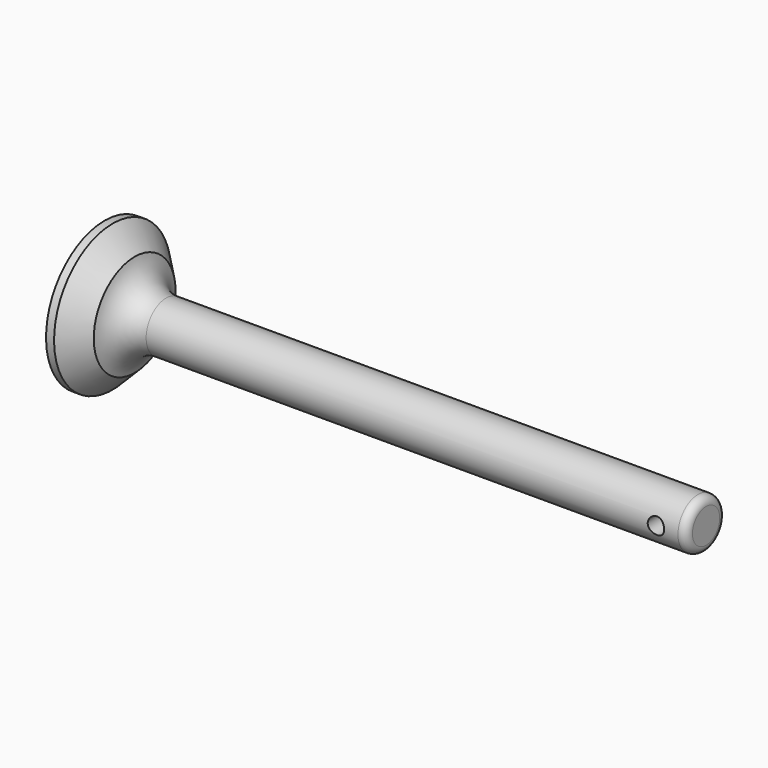
from build123d import *

# Parameters (mm, degrees)
F3_R     = 0.508
F6_R     = 0.5207
F7_DEPTH = 9.7165


# Not quite as in the source:
# - a fillet or chamfer that OpenCascade refuses, or shapes differently, is made with other operations: its cross-section is extruded or revolved along the edge and cut away or added


with BuildPart() as f1:
    # F0 (on Front) → F1 (revolve)
    with BuildSketch(Plane.XZ):
        Polygon((0, 4.6355), (0, 0), (38.1, 0), (38.1, 1.5875), (1.905, 1.5875), (1.905, 3.2385), (0.508, 4.6355), align=None)
    revolve(axis=Axis((19.05, 0, 0), (1, 0, 0)))

    # F2: fillet of radius 2.032 on 1 edges, made by hand

    # F2_s1 → F2_t2 (revolve)
    with BuildSketch(Plane.XZ):
        with BuildLine():
            ThreePointArc((1.905, 3.2385), (2.6058107165, 2.0537388432), (3.900961673, 1.5875))
            Line((3.900961673, 1.5875), (3.900961673, 1.54686))
            Line((3.900961673, 1.54686), (1.905, 1.54686))
            Line((1.905, 1.54686), (1.86436, 1.5875))
            ThreePointArc((1.86436, 1.5875), (1.86436, 2.413), (1.8650807665, 3.23088))
            Line((1.8650807665, 3.23088), (1.905, 3.2385))
        make_face()
    revolve(axis=Axis((1.905, 0, 0), (1, 0, 0)))

    # F3
    f3_edges = [f1.edges().sort_by_distance(p)[0] for p in [
        (38.1, 0, -1.5875),
    ]]
    fillet(f3_edges, radius=F3_R)

    # F6 (on offset) → F7 (cut, through all)
    with BuildSketch(Plane.XZ.offset(5.08)):
        with Locations((36.195, 0)):
            Circle(F6_R)
    extrude(amount=-F7_DEPTH, mode=Mode.SUBTRACT)


solid = f1.part
